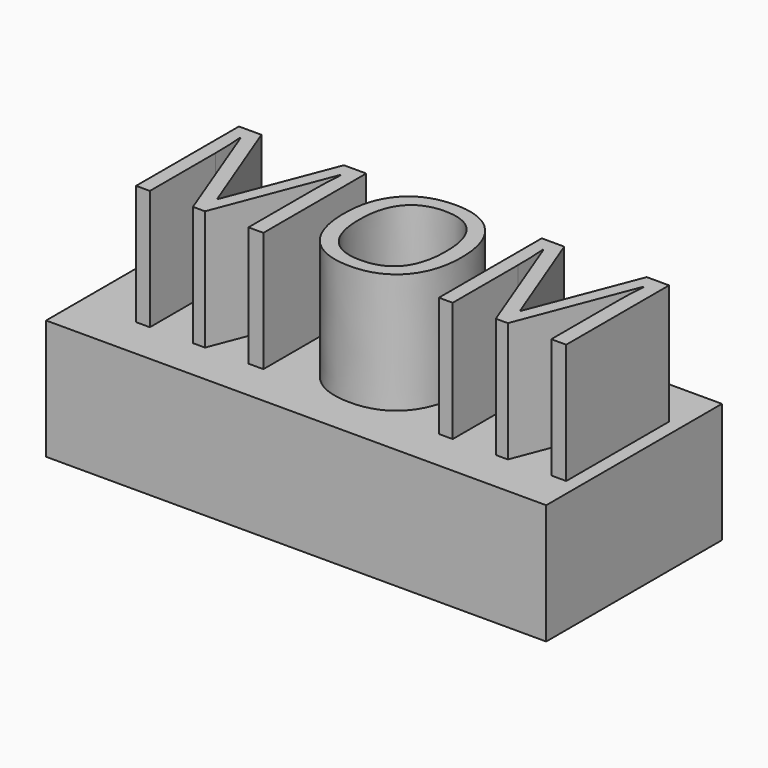
from build123d import *

# Parameters (mm, degrees)
F0_W         = 80.4569832981
F0_H         = 46.486256877
F1_DEPTH     = 25.4
F2_TEXT_SIZE = 38.1159188692
F3_DEPTH     = 25.4
F5_DEPTH     = 25.4


# Not quite as in the source:
# - Text() gives the source's letters only with a copy of the font that has no kerning and outlines rounded to 1/6400 em; it was checked with that copy


with BuildPart() as f1:
    # F0 (on Top) → F1 (new body)
    with BuildSketch(Plane.XY):
        with Locations((-5.065811798, 19.5182681782)):
            Rectangle(F0_W, F0_H)
    extrude(amount=F1_DEPTH)

    # F2 (on face) → F3 (join)
    with BuildSketch(Plane.XY.offset(25.4)):
        with Locations((-37.0532236993, 5.1056216471)):
            Text('MOM', F2_TEXT_SIZE, font='Open Sans', text_align=(TextAlign.LEFT, TextAlign.BOTTOM))
    extrude(amount=F3_DEPTH)

    # F4 (on face) → F5 (join)
    with BuildSketch(Plane.YZ.offset(35.1626798511)):
        Polygon((25.1224694959, 25.4), (-3.7248602603, 25.4), (-3.7248602603, 0), (42.7613966167, 0), (42.7613966167, 25.4), (32.3168143523, 25.4), align=None)
    extrude(amount=F5_DEPTH)


solid = f1.part
